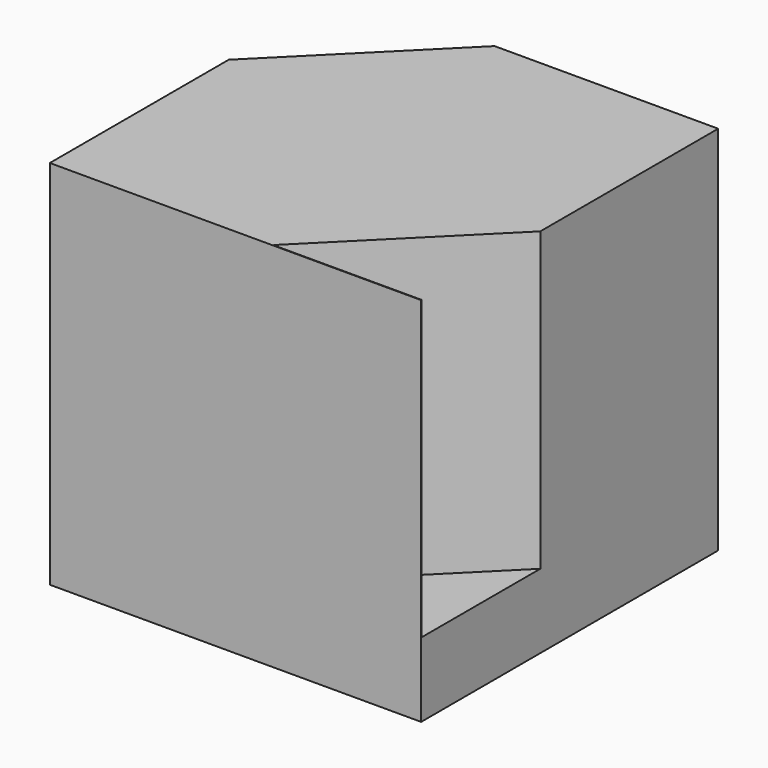
from build123d import *

# Parameters (mm, degrees)
F0_W     = 127
F0_H     = 127
F1_DEPTH = 127
F3_DEPTH = 101.6


# Not quite as in the source:
# - a feature names something its author has since deleted; it is built from what else it names


with BuildPart() as f1:
    # F0 (on Top) → F1 (new body)
    with BuildSketch(Plane.XY):
        Rectangle(F0_W, F0_H)
    extrude(amount=-F1_DEPTH)

    # F2 (on Top) → F3 (cut)
    with BuildSketch(Plane.XY):
        Polygon((-12.9577365428, 63.5224819239), (-63.7577365428, 63.5224819239), (-63.7577365428, 12.7224819239), align=None)
        Polygon((12.7373517871, -63.3020326495), (63.5373517871, -63.3020326495), (63.5373517871, -12.5020326495), align=None)
    extrude(amount=-F3_DEPTH, mode=Mode.SUBTRACT)


solid = f1.part
